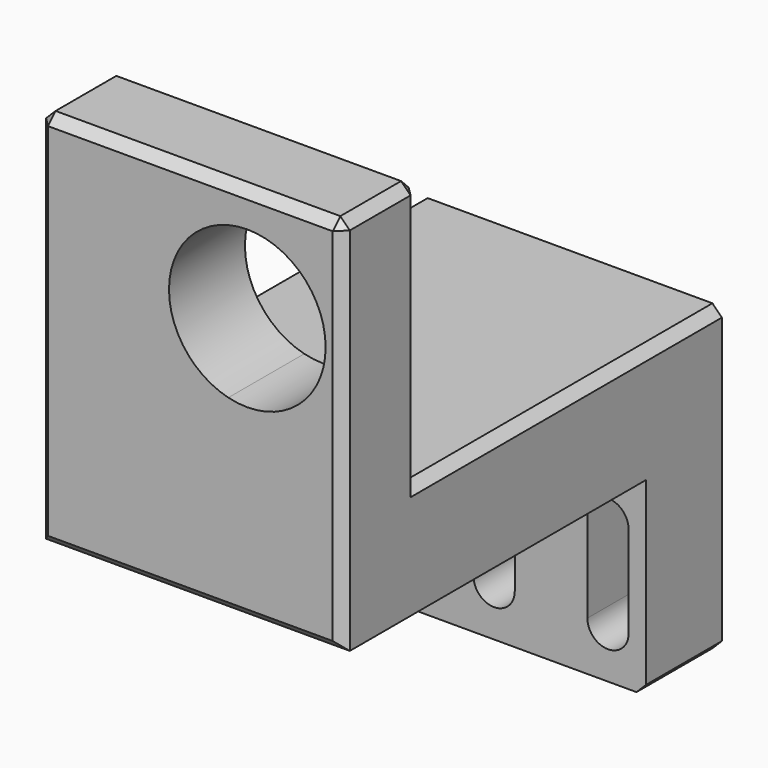
from build123d import *

# Parameters (mm, degrees)
F1_DEPTH = 50
F2_W     = 40
F2_H     = 28
F2_H_2   = 20
F3_DEPTH = 32.001
F4_SIZE  = 1


with BuildPart() as f1:
    # F0 (on Front) → F1 (new body)
    with BuildSketch(Plane.XZ):
        with BuildLine():
            Line((-22, 30), (-22, -30))
            Line((-22, -30), (-2, -30))
            Line((-2, -30), (-2, 9.9960947032))
            ThreePointArc((-2, 9.9960947032), (-8.25, 18), (-2, 26.0039052968))
            Line((-2, 26.0039052968), (-2, 30))
            Line((-2, 30), (-22, 30))
        make_face()
        with BuildLine():
            ThreePointArc((-15.825, -24.825), (-18, -27), (-20.175, -24.825))
            Line((-20.175, -24.825), (-20.175, -15.175))
            ThreePointArc((-20.175, -15.175), (-18, -13), (-15.825, -15.175))
            Line((-15.825, -15.175), (-15.825, -24.825))
        make_face(mode=Mode.SUBTRACT)
        with BuildLine():
            ThreePointArc((-3.825, -24.825), (-6, -27), (-8.175, -24.825))
            Line((-8.175, -24.825), (-8.175, -15.175))
            ThreePointArc((-8.175, -15.175), (-6, -13), (-3.825, -15.175))
            Line((-3.825, -15.175), (-3.825, -24.825))
        make_face(mode=Mode.SUBTRACT)
        with BuildLine():
            Line((-2, 9.9960947032), (-2, -30))
            Line((-2, -30), (10, -30))
            Line((10, -30), (10, 30))
            Line((10, 30), (-2, 30))
            Line((-2, 30), (-2, 26.0039052968))
            ThreePointArc((-2, 26.0039052968), (5.0775240029, 24.5024034018), (8.25, 18))
            ThreePointArc((8.25, 18), (5.0775240029, 11.4975965982), (-2, 9.9960947032))
        make_face()
        with BuildLine():
            Line((3.825, -24.825), (3.825, -15.175))
            ThreePointArc((3.825, -15.175), (6, -13), (8.175, -15.175))
            Line((8.175, -15.175), (8.175, -24.825))
            ThreePointArc((8.175, -24.825), (6, -27), (3.825, -24.825))
        make_face(mode=Mode.SUBTRACT)
    extrude(amount=F1_DEPTH)

    # F2 (on face) → F3 (cut, through all)
    with BuildSketch(Plane.YZ.offset(10)):
        with Locations((-20, 16)):
            Rectangle(F2_W, F2_H)
        with Locations((-30, -20)):
            Rectangle(F2_W, F2_H_2)
    extrude(amount=-F3_DEPTH, mode=Mode.SUBTRACT)

    # F4
    f4_edges = [f1.edges().sort_by_distance(p)[0] for p in [
        (10, -20, 2),
        (10, -40, 16),
        (10, -45, 30),
        (10, -50, 10),
        (10, -5, -30),
        (-6, -50, 30),
        (-22, -20, 2),
        (-22, -5, -30),
        (-22, -50, 10),
        (-22, -45, 30),
        (-22, -40, 16),
        (-6, -50, -10),
        (-6, -40, 30),
    ]]
    chamfer(f4_edges, length=F4_SIZE)


solid = f1.part
